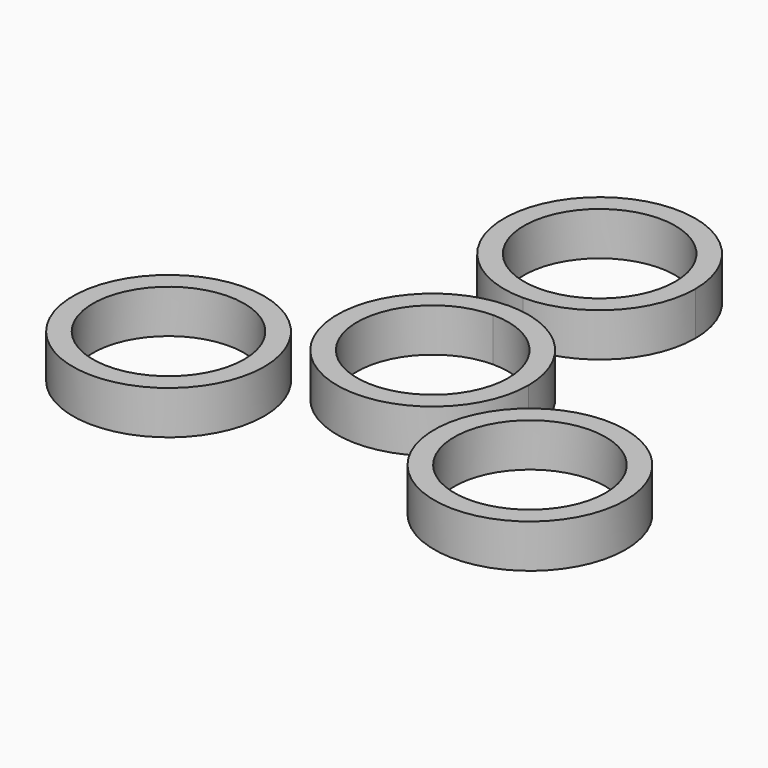
from build123d import *

# Parameters (mm, degrees)
F2_DEPTH = 6.35
F0_R     = 13.97
F0_R_2   = 11.049


# Not quite as in the source:
# - the program builds the solid bodies; features that only make, move or delete a surface that nothing else refers to are left out


with BuildPart() as f2:
    # F0 (on Top) → F2 (new body)
    with BuildSketch(Plane.XY):
        with BuildLine():
            ThreePointArc((13.97, 30.48), (-9.8782817332, 40.3582817332), (0, 16.51))
            ThreePointArc((0, 16.51), (9.8782817332, 20.6017182668), (13.97, 30.48))
        make_face()
        with BuildLine():
            ThreePointArc((11.049, 30.48), (7.8128228253, 22.6671771747), (0, 19.431))
            ThreePointArc((0, 19.431), (-7.8128228253, 38.2928228253), (11.049, 30.48))
        make_face(mode=Mode.SUBTRACT)
    extrude(amount=F2_DEPTH)


with BuildPart() as f2b:
    # F0 (on Top) → F2, piece 2 (new body)
    with BuildSketch(Plane.XY):
        with Locations((-26.3964543073, -15.24)):
            Circle(F0_R)
        with Locations((-26.3964543073, -15.24)):
            Circle(F0_R_2, mode=Mode.SUBTRACT)
    extrude(amount=F2_DEPTH)


with BuildPart() as f2c:
    # F0 (on Top) → F2, piece 3 (new body)
    with BuildSketch(Plane.XY):
        with Locations((26.3964543073, -15.24)):
            Circle(F0_R)
        with Locations((26.3964543073, -15.24)):
            Circle(F0_R_2, mode=Mode.SUBTRACT)
    extrude(amount=F2_DEPTH)


with BuildPart() as f2d:
    # F0 (on Top) → F2, piece 4 (new body)
    with BuildSketch(Plane.XY):
        with BuildLine():
            ThreePointArc((13.97, 0), (9.8782817332, 9.8782817332), (0, 13.97))
            ThreePointArc((0, 13.97), (-9.8782817332, -9.8782817332), (13.97, 0))
        make_face()
        with BuildLine():
            ThreePointArc((0, 11.049), (7.8128228253, 7.8128228253), (11.049, 0))
            ThreePointArc((11.049, 0), (-7.8128228253, -7.8128228253), (0, 11.049))
        make_face(mode=Mode.SUBTRACT)
    extrude(amount=F2_DEPTH)


solid = Compound([f2.part, f2b.part, f2c.part, f2d.part])
